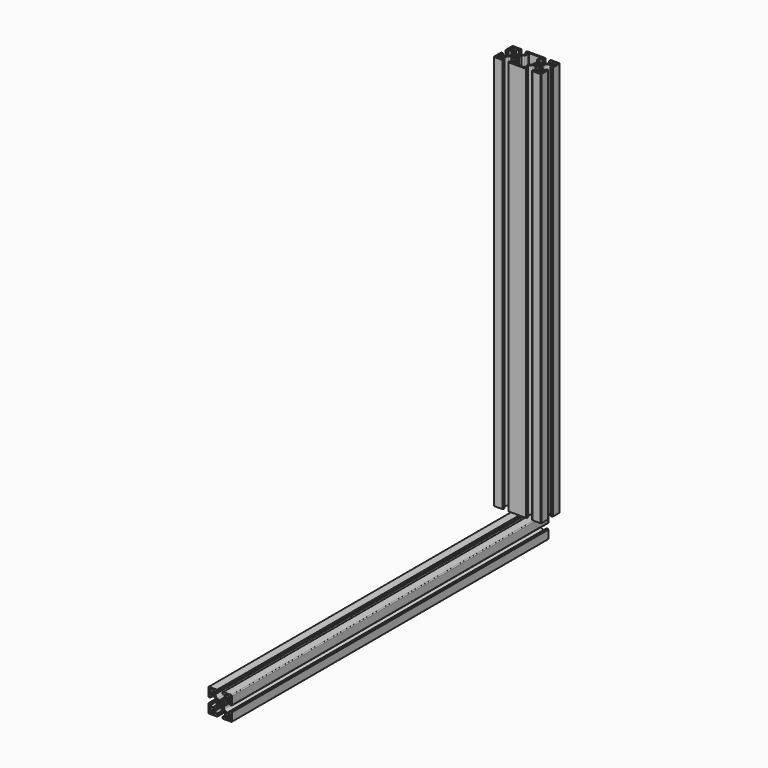
from build123d import *

# Parameters (mm, degrees)
F2_DEPTH = 500
F3_DEPTH = 500


# Not quite as in the source:
# - ends of sketch curves that miss each other by under 0.0002 mm in the source are joined


with BuildPart() as f2:
    # F1 (on Front) → F2 (new body)
    with BuildSketch(Plane.XZ):
        with BuildLine():
            Line((-16.817882, -28.053804), (-15.317882, -28.053804))
            ThreePointArc((-15.317882, -28.053804), (-15.2613573135, -27.5251941322), (-15.0943392862, -27.0204878701))
            ThreePointArc((-15.0943392862, -27.0204878701), (-15.1018556445, -26.757114112), (-15.3142900125, -26.6012490693))
            Line((-15.3142900125, -26.6012490693), (-16.055223, -26.467679))
            ThreePointArc((-16.055223, -26.467679), (-16.2747726412, -26.2973161033), (-16.2602657097, -26.0198001716))
            ThreePointArc((-16.2602657097, -26.0198001716), (-15.6451391247, -25.2265468753), (-14.8518861678, -24.611419716))
            ThreePointArc((-14.8518861678, -24.611419716), (-14.574370128, -24.5969122529), (-14.4040070693, -24.8164620125))
            Line((-14.4040070693, -24.8164620125), (-14.270436, -25.557396))
            ThreePointArc((-14.270436, -25.557396), (-14.114570705, -25.7698304515), (-13.8511966819, -25.7773467007))
            ThreePointArc((-13.8511966819, -25.7773467007), (-13.3464912208, -25.6103285465), (-12.817882, -25.553804))
            Line((-12.817882, -25.553804), (-12.817882, -24.053804))
            Line((-12.817882, -24.053804), (-13.317882, -23.553804))
            Line((-13.317882, -23.553804), (-15.035723, -23.553804))
            ThreePointArc((-15.035723, -23.553804), (-15.9762206131, -23.4025693887), (-16.8218943655, -22.9641134932))
            ThreePointArc((-16.8218943655, -22.9641134932), (-18.0925440917, -21.1637239049), (-18.9312372647, -19.1259440756))
            ThreePointArc((-18.9312372647, -19.1259440756), (-18.952848093, -18.864054156), (-18.9054896298, -18.6055767962))
            Line((-18.9054896298, -18.6055767962), (-17.917882, -15.553804))
            Line((-17.917882, -15.553804), (-16.267882, -15.553804))
            ThreePointArc((-16.267882, -15.553804), (-16.0557499656, -15.4659360344), (-15.967882, -15.253804))
            Line((-15.967882, -15.253804), (-15.967882, -13.553804))
            Line((-15.967882, -13.553804), (-16.767882, -13.053804))
            Line((-16.767882, -13.053804), (-26.817882, -13.053804))
            ThreePointArc((-26.817882, -13.053804), (-27.5249887812, -13.3466972188), (-27.817882, -14.053804))
            Line((-27.817882, -14.053804), (-27.817882, -24.103804))
            Line((-27.817882, -24.103804), (-27.317882, -24.903804))
            Line((-27.317882, -24.903804), (-25.617882, -24.903804))
            ThreePointArc((-25.617882, -24.903804), (-25.4057499656, -24.8159360344), (-25.317882, -24.603804))
            Line((-25.317882, -24.603804), (-25.317882, -22.953804))
            Line((-25.317882, -22.953804), (-22.266108, -21.966196))
            ThreePointArc((-22.266108, -21.966196), (-22.0076307271, -21.9188378518), (-21.7457409226, -21.9404486442))
            ThreePointArc((-21.7457409226, -21.9404486442), (-19.7079616374, -22.7791421598), (-17.907572504, -24.049791567))
            ThreePointArc((-17.907572504, -24.049791567), (-17.4691166439, -24.8954652882), (-17.317882, -25.835963))
            Line((-17.317882, -25.835963), (-17.317882, -27.553804))
            Line((-17.317882, -27.553804), (-16.817882, -28.053804))
        make_face()
        with BuildLine():
            ThreePointArc((-20.1318415243, -16.7176952608), (-19.817882, -18.053804), (-20.1318415243, -19.3899127392))
            ThreePointArc((-20.1318415243, -19.3899127392), (-20.1593135799, -19.5718836819), (-20.0753690344, -19.7356560344))
            Line((-20.0753690344, -19.7356560344), (-19.334799, -20.476227))
            ThreePointArc((-19.334799, -20.476227), (-19.2473630595, -20.6722640002), (-19.3132911489, -20.8765408801))
            ThreePointArc((-19.3132911489, -20.8765408801), (-19.6359009875, -21.2357840182), (-19.9951440617, -21.5583939234))
            ThreePointArc((-19.9951440617, -21.5583939234), (-20.1994212978, -21.6243229782), (-20.3954590344, -21.5368870344))
            Line((-20.3954590344, -21.5368870344), (-21.136029, -20.796316))
            ThreePointArc((-21.136029, -20.796316), (-21.2998015274, -20.7123715492), (-21.4817721923, -20.7398436134))
            ThreePointArc((-21.4817721923, -20.7398436134), (-22.8178815523, -21.053804), (-24.153991138, -20.7398442773))
            ThreePointArc((-24.153991138, -20.7398442773), (-24.3359616819, -20.7123714201), (-24.4997340344, -20.7963159656))
            Line((-24.4997340344, -20.7963159656), (-25.240304, -21.536887))
            ThreePointArc((-25.240304, -21.536887), (-25.4363417022, -21.6243229782), (-25.6406189751, -21.5583939691))
            ThreePointArc((-25.6406189751, -21.5583939691), (-25.9998625153, -21.2357845153), (-26.322472412, -20.8765413318))
            ThreePointArc((-26.322472412, -20.8765413318), (-26.3884009573, -20.6722643134), (-26.3009650344, -20.4762269656))
            Line((-26.3009650344, -20.4762269656), (-25.560394, -19.735656))
            ThreePointArc((-25.560394, -19.735656), (-25.4764494201, -19.5718836819), (-25.5039220121, -19.389913006))
            ThreePointArc((-25.5039220121, -19.389913006), (-25.817882, -18.053804), (-25.5039222773, -16.717694862))
            ThreePointArc((-25.5039222773, -16.717694862), (-25.4764494201, -16.5357243181), (-25.5603939656, -16.3719519656))
            Line((-25.5603939656, -16.3719519656), (-26.300965, -15.631381))
            ThreePointArc((-26.300965, -15.631381), (-26.3884009573, -15.4353436866), (-26.3224724576, -15.2310666314))
            ThreePointArc((-26.3224724576, -15.2310666314), (-25.9998625153, -14.8718234847), (-25.6406193318, -14.549213588))
            ThreePointArc((-25.6406193318, -14.549213588), (-25.4363417022, -14.4832850218), (-25.2403039656, -14.5707209656))
            Line((-25.2403039656, -14.5707209656), (-24.499734, -15.311292))
            ThreePointArc((-24.499734, -15.311292), (-24.3359616819, -15.3952365799), (-24.153991006, -15.3677639879))
            ThreePointArc((-24.153991006, -15.3677639879), (-22.8178815523, -15.053804), (-21.4817720604, -15.3677641214))
            ThreePointArc((-21.4817720604, -15.3677641214), (-21.2998015274, -15.3952364508), (-21.1360294656, -15.3112915344))
            Line((-21.1360294656, -15.3112915344), (-20.395459, -14.570721))
            ThreePointArc((-20.395459, -14.570721), (-20.1994212978, -14.4832850218), (-19.9951440249, -14.5492140309))
            ThreePointArc((-19.9951440249, -14.5492140309), (-19.6359009875, -14.8718239818), (-19.3132911946, -15.2310671567))
            ThreePointArc((-19.3132911946, -15.2310671567), (-19.2473630595, -15.4353439998), (-19.3347989656, -15.6313810344))
            Line((-19.3347989656, -15.6313810344), (-20.075369, -16.371952))
            ThreePointArc((-20.075369, -16.371952), (-20.1593135799, -16.5357243181), (-20.1318415243, -16.7176952608))
        make_face(mode=Mode.SUBTRACT)
        with BuildLine():
            Line((-10.317882, -28.053804), (-8.817882, -28.053804))
            Line((-8.817882, -28.053804), (-8.317882, -27.553804))
            Line((-8.317882, -27.553804), (-8.317882, -25.835963))
            ThreePointArc((-8.317882, -25.835963), (-8.1666472628, -24.8954650055), (-7.7281910149, -24.049790989))
            ThreePointArc((-7.7281910149, -24.049790989), (-5.9278016138, -22.7791417483), (-3.8900220756, -21.9404487353))
            ThreePointArc((-3.8900220756, -21.9404487353), (-3.6281322729, -21.9188378518), (-3.3696549943, -21.9661959825))
            Line((-3.3696549943, -21.9661959825), (-0.317882, -22.953804))
            Line((-0.317882, -22.953804), (-0.317882, -24.603804))
            ThreePointArc((-0.317882, -24.603804), (-0.2300140344, -24.8159360344), (-0.017882, -24.903804))
            Line((-0.017882, -24.903804), (1.682118, -24.903804))
            Line((1.682118, -24.903804), (2.182118, -24.103804))
            Line((2.182118, -24.103804), (2.182118, -14.053804))
            ThreePointArc((2.182118, -14.053804), (1.8892247812, -13.3466972188), (1.182118, -13.053804))
            Line((1.182118, -13.053804), (-8.867882, -13.053804))
            Line((-8.867882, -13.053804), (-9.667882, -13.553804))
            Line((-9.667882, -13.553804), (-9.667882, -15.253804))
            ThreePointArc((-9.667882, -15.253804), (-9.5800140344, -15.4659360344), (-9.367882, -15.553804))
            Line((-9.367882, -15.553804), (-7.717882, -15.553804))
            Line((-7.717882, -15.553804), (-6.730274, -18.605577))
            ThreePointArc((-6.730274, -18.605577), (-6.6829159047, -18.8640542036), (-6.7045263914, -19.1259439149))
            ThreePointArc((-6.7045263914, -19.1259439149), (-7.5432189083, -21.1637239049), (-8.8138685119, -22.9641134339))
            ThreePointArc((-8.8138685119, -22.9641134339), (-9.6595430055, -23.4025692628), (-10.600041, -23.553804))
            Line((-10.600041, -23.553804), (-12.317882, -23.553804))
            Line((-12.317882, -23.553804), (-12.817882, -24.053804))
            Line((-12.817882, -24.053804), (-12.817882, -25.553804))
            ThreePointArc((-12.817882, -25.553804), (-12.2892723342, -25.6103286428), (-11.7845662465, -25.777346543))
            ThreePointArc((-11.7845662465, -25.777346543), (-11.521192295, -25.7698304515), (-11.3653270693, -25.5573959875))
            Line((-11.3653270693, -25.5573959875), (-11.231756, -24.816462))
            ThreePointArc((-11.231756, -24.816462), (-11.061392872, -24.5969122529), (-10.7838767336, -24.6114195492))
            ThreePointArc((-10.7838767336, -24.6114195492), (-9.990624391, -25.2265473595), (-9.3754974572, -26.0198002702))
            ThreePointArc((-9.3754974572, -26.0198002702), (-9.3609903588, -26.2973161033), (-9.5805400125, -26.4676789307))
            Line((-9.5805400125, -26.4676789307), (-10.321473, -26.601249))
            ThreePointArc((-10.321473, -26.601249), (-10.5339073555, -26.757114112), (-10.5414238716, -27.0204879417))
            ThreePointArc((-10.5414238716, -27.0204879417), (-10.3744066428, -27.5251943342), (-10.317882, -28.053804))
        make_face()
        with BuildLine():
            ThreePointArc((-5.5627339656, -19.7356560344), (-5.4787894201, -19.5718836819), (-5.5062620121, -19.389913006))
            ThreePointArc((-5.5062620121, -19.389913006), (-5.820221, -18.053804), (-5.5062614757, -16.7176952608))
            ThreePointArc((-5.5062614757, -16.7176952608), (-5.4787894201, -16.5357243181), (-5.5627339656, -16.3719519656))
            Line((-5.5627339656, -16.3719519656), (-6.303305, -15.631381))
            ThreePointArc((-6.303305, -15.631381), (-6.3907399595, -15.4353436467), (-6.3248118511, -15.2310671199))
            ThreePointArc((-6.3248118511, -15.2310671199), (-6.0022020125, -14.8718239818), (-5.6429589383, -14.5492140766))
            ThreePointArc((-5.6429589383, -14.5492140766), (-5.4386817022, -14.4832850218), (-5.2426439656, -14.5707209656))
            Line((-5.2426439656, -14.5707209656), (-4.502074, -15.311292))
            ThreePointArc((-4.502074, -15.311292), (-4.3383016819, -15.3952365799), (-4.156331006, -15.3677639879))
            ThreePointArc((-4.156331006, -15.3677639879), (-2.8202214477, -15.053804), (-1.484111862, -15.3677637227))
            ThreePointArc((-1.484111862, -15.3677637227), (-1.3021413181, -15.3952365799), (-1.1383689656, -15.3112920344))
            Line((-1.1383689656, -15.3112920344), (-0.397799, -14.570721))
            ThreePointArc((-0.397799, -14.570721), (-0.2017612978, -14.4832850218), (0.0025159751, -14.5492140309))
            ThreePointArc((0.0025159751, -14.5492140309), (0.3617595153, -14.8718234847), (0.684369412, -15.2310666682))
            ThreePointArc((0.684369412, -15.2310666682), (0.7502979573, -15.4353436866), (0.6628620344, -15.6313810344))
            Line((0.6628620344, -15.6313810344), (-0.077709, -16.371952))
            ThreePointArc((-0.077709, -16.371952), (-0.1616535799, -16.5357243181), (-0.1341809879, -16.717694994))
            ThreePointArc((-0.1341809879, -16.717694994), (0.179779, -18.053804), (-0.1341807227, -19.389913138))
            ThreePointArc((-0.1341807227, -19.389913138), (-0.1616535799, -19.5718836819), (-0.0777090344, -19.7356560344))
            Line((-0.0777090344, -19.7356560344), (0.662862, -20.476227))
            ThreePointArc((0.662862, -20.476227), (0.7502979573, -20.6722643134), (0.6843694576, -20.8765413686))
            ThreePointArc((0.6843694576, -20.8765413686), (0.3617595153, -21.2357845153), (0.0025163318, -21.558394412))
            ThreePointArc((0.0025163318, -21.558394412), (-0.2017612978, -21.6243229782), (-0.3977990344, -21.5368870344))
            Line((-0.3977990344, -21.5368870344), (-1.138369, -20.796316))
            ThreePointArc((-1.138369, -20.796316), (-1.3021413181, -20.7123714201), (-1.484111994, -20.7398440121))
            ThreePointArc((-1.484111994, -20.7398440121), (-2.8202214477, -21.053804), (-4.1563309396, -20.7398438786))
            ThreePointArc((-4.1563309396, -20.7398438786), (-4.3383016819, -20.7123714201), (-4.5020740344, -20.7963159656))
            Line((-4.5020740344, -20.7963159656), (-5.242644, -21.536887))
            ThreePointArc((-5.242644, -21.536887), (-5.4386817022, -21.6243229782), (-5.6429589751, -21.5583939691))
            ThreePointArc((-5.6429589751, -21.5583939691), (-6.0022020125, -21.2357840182), (-6.3248118054, -20.8765408433))
            ThreePointArc((-6.3248118054, -20.8765408433), (-6.3907399595, -20.6722643533), (-6.3033045344, -20.4762274656))
            Line((-6.3033045344, -20.4762274656), (-5.5627339656, -19.7356560344))
        make_face(mode=Mode.SUBTRACT)
        with BuildLine():
            Line((-8.317882, -28.553804), (-8.817882, -28.053804))
            Line((-8.817882, -28.053804), (-10.317882, -28.053804))
            ThreePointArc((-10.317882, -28.053804), (-10.3744066428, -28.5824136658), (-10.541424543, -29.0871197535))
            ThreePointArc((-10.541424543, -29.0871197535), (-10.5339073967, -29.3504938095), (-10.3214731621, -29.5063588992))
            Line((-10.3214731621, -29.5063588992), (-9.58054, -29.639929))
            ThreePointArc((-9.58054, -29.639929), (-9.3609903588, -29.8102918967), (-9.3754972903, -30.0878078284))
            ThreePointArc((-9.3754972903, -30.0878078284), (-9.990624391, -30.8810606405), (-10.783877091, -31.496187846))
            ThreePointArc((-10.783877091, -31.496187846), (-11.061392872, -31.5106957471), (-11.2317559307, -31.2911459875))
            Line((-11.2317559307, -31.2911459875), (-11.365327, -30.550212))
            ThreePointArc((-11.365327, -30.550212), (-11.521192112, -30.3377776445), (-11.7845659417, -30.3302611284))
            ThreePointArc((-11.7845659417, -30.3302611284), (-12.2892721322, -30.4972793135), (-12.817882, -30.553804))
            Line((-12.817882, -30.553804), (-12.817882, -32.053804))
            Line((-12.817882, -32.053804), (-12.317882, -32.553804))
            Line((-12.317882, -32.553804), (-10.600041, -32.553804))
            ThreePointArc((-10.600041, -32.553804), (-9.6595430055, -32.7050387372), (-8.813868989, -33.1434949851))
            ThreePointArc((-8.813868989, -33.1434949851), (-7.5432189083, -34.9438840951), (-6.7045257353, -36.9816639244))
            ThreePointArc((-6.7045257353, -36.9816639244), (-6.6829158812, -37.2435533212), (-6.7302739825, -37.5020300057))
            Line((-6.7302739825, -37.5020300057), (-7.717882, -40.553804))
            Line((-7.717882, -40.553804), (-9.367882, -40.553804))
            ThreePointArc((-9.367882, -40.553804), (-9.5800140344, -40.6416719656), (-9.667882, -40.853804))
            Line((-9.667882, -40.853804), (-9.667882, -42.553804))
            Line((-9.667882, -42.553804), (-8.867882, -43.053804))
            Line((-8.867882, -43.053804), (1.182118, -43.053804))
            ThreePointArc((1.182118, -43.053804), (1.8892247812, -42.7609107812), (2.182118, -42.053804))
            Line((2.182118, -42.053804), (2.182118, -32.003804))
            Line((2.182118, -32.003804), (1.682118, -31.203804))
            Line((1.682118, -31.203804), (-0.017882, -31.203804))
            ThreePointArc((-0.017882, -31.203804), (-0.2300140344, -31.2916719656), (-0.317882, -31.503804))
            Line((-0.317882, -31.503804), (-0.317882, -33.153804))
            Line((-0.317882, -33.153804), (-3.369655, -34.141412))
            ThreePointArc((-3.369655, -34.141412), (-3.6281322729, -34.1887701482), (-3.8900220774, -34.1671593558))
            ThreePointArc((-3.8900220774, -34.1671593558), (-5.9278016138, -33.3284662517), (-7.7281909374, -32.0578169295))
            ThreePointArc((-7.7281909374, -32.0578169295), (-8.1666472628, -31.2121429945), (-8.317882, -30.271645))
            Line((-8.317882, -30.271645), (-8.317882, -28.553804))
        make_face()
        with BuildLine():
            ThreePointArc((-5.507146239, -39.3904841188), (-5.8210019909, -38.0543501064), (-5.5069379006, -36.7182650494))
            ThreePointArc((-5.5069379006, -36.7182650494), (-5.4794506299, -36.5362965287), (-5.5633824662, -36.3725174663))
            Line((-5.5633824662, -36.3725174663), (-6.303896, -35.631889))
            ThreePointArc((-6.303896, -35.631889), (-6.3913162338, -35.4358449105), (-6.3253716664, -35.2315732687))
            ThreePointArc((-6.3253716664, -35.2315732687), (-6.0027340882, -34.8723550769), (-5.6434657786, -34.5497732749))
            ThreePointArc((-5.6434657786, -34.5497732749), (-5.4391833549, -34.483860277), (-5.2431524662, -34.5713114663))
            Line((-5.2431524662, -34.5713114663), (-4.50264, -35.31194))
            ThreePointArc((-4.50264, -35.31194), (-4.3388740212, -35.3958977668), (-4.1569008286, -35.3684393446))
            ThreePointArc((-4.1569008286, -35.3684393446), (-2.8207674361, -35.0545840092), (-1.4846830494, -35.3686480994))
            ThreePointArc((-1.4846830494, -35.3686480994), (-1.3027146578, -35.3961343911), (-1.1389359663, -35.3122030337))
            Line((-1.1389359663, -35.3122030337), (-0.398307, -34.57169))
            ThreePointArc((-0.398307, -34.57169), (-0.2022626922, -34.4842688081), (0.0020096134, -34.5502132386))
            ThreePointArc((0.0020096134, -34.5502132386), (0.3612269231, -34.8728519118), (0.6838087251, -35.2321202214))
            ThreePointArc((0.6838087251, -35.2321202214), (0.7497216831, -35.4364023869), (0.6622700337, -35.6324330337))
            Line((0.6622700337, -35.6324330337), (-0.078358, -36.372946))
            ThreePointArc((-0.078358, -36.372946), (-0.1623158238, -36.5367113277), (-0.1348573446, -36.7186841714))
            ThreePointArc((-0.1348573446, -36.7186841714), (0.1789979909, -38.0548178935), (-0.1350659009, -39.3909025518))
            ThreePointArc((-0.1350659009, -39.3909025518), (-0.162552241, -39.5728712621), (-0.0786200338, -39.7366500338))
            Line((-0.0786200338, -39.7366500338), (0.661893, -40.477278))
            ThreePointArc((0.661893, -40.477278), (0.7493132149, -40.6733227364), (0.6833686664, -40.8775947313))
            ThreePointArc((0.6833686664, -40.8775947313), (0.3607308072, -41.2368122042), (0.0014628737, -41.5593938432))
            ThreePointArc((0.0014628737, -41.5593938432), (-0.202819292, -41.625306742), (-0.3988500338, -41.5378560338))
            Line((-0.3988500338, -41.5378560338), (-1.139363, -40.797227))
            ThreePointArc((-1.139363, -40.797227), (-1.303129108, -40.7132702121), (-1.4851017727, -40.7407284571))
            ThreePointArc((-1.4851017727, -40.7407284571), (-2.8212354459, -41.0545839909), (-4.157320149, -40.7405202994))
            ThreePointArc((-4.157320149, -40.7405202994), (-4.3392886912, -40.7130336658), (-4.5030675338, -40.7969654663))
            Line((-4.5030675338, -40.7969654663), (-5.243696, -41.537478))
            ThreePointArc((-5.243696, -41.537478), (-5.4397403476, -41.624898194), (-5.6440121248, -41.5589541549))
            ThreePointArc((-5.6440121248, -41.5589541549), (-6.0032304261, -41.2363165853), (-6.3258123317, -40.8770482671))
            ThreePointArc((-6.3258123317, -40.8770482671), (-6.3917246831, -40.6727656131), (-6.3042730337, -40.4767349663))
            Line((-6.3042730337, -40.4767349663), (-5.563645, -39.736222))
            ThreePointArc((-5.563645, -39.736222), (-5.4796873054, -39.5724564631), (-5.507146239, -39.3904841188))
        make_face(mode=Mode.SUBTRACT)
        with BuildLine():
            ThreePointArc((-15.0943392862, -29.0871201299), (-15.2613573135, -28.5824138678), (-15.317882, -28.053804))
            Line((-15.317882, -28.053804), (-16.817882, -28.053804))
            Line((-16.817882, -28.053804), (-17.317882, -28.553804))
            Line((-17.317882, -28.553804), (-17.317882, -30.271645))
            ThreePointArc((-17.317882, -30.271645), (-17.4691166439, -31.2121427118), (-17.9075726307, -32.0578165326))
            ThreePointArc((-17.9075726307, -32.0578165326), (-19.7079616374, -33.3284658402), (-21.7457409999, -34.1671590005))
            ThreePointArc((-21.7457409999, -34.1671590005), (-22.0076307271, -34.1887701482), (-22.2661080057, -34.1414120175))
            Line((-22.2661080057, -34.1414120175), (-25.317882, -33.153804))
            Line((-25.317882, -33.153804), (-25.317882, -31.503804))
            ThreePointArc((-25.317882, -31.503804), (-25.4057499656, -31.2916719656), (-25.617882, -31.203804))
            Line((-25.617882, -31.203804), (-27.317882, -31.203804))
            Line((-27.317882, -31.203804), (-27.817882, -32.003804))
            Line((-27.817882, -32.003804), (-27.817882, -42.053804))
            ThreePointArc((-27.817882, -42.053804), (-27.5249887812, -42.7609107812), (-26.817882, -43.053804))
            Line((-26.817882, -43.053804), (-16.767882, -43.053804))
            Line((-16.767882, -43.053804), (-15.967882, -42.553804))
            Line((-15.967882, -42.553804), (-15.967882, -40.853804))
            ThreePointArc((-15.967882, -40.853804), (-16.0557499656, -40.6416719656), (-16.267882, -40.553804))
            Line((-16.267882, -40.553804), (-17.917882, -40.553804))
            Line((-17.917882, -40.553804), (-18.905489, -37.50203))
            ThreePointArc((-18.905489, -37.50203), (-18.9528481165, -37.2435533689), (-18.9312375634, -36.9816638775))
            ThreePointArc((-18.9312375634, -36.9816638775), (-18.0925440917, -34.9438840951), (-16.8218944881, -33.1434945661))
            ThreePointArc((-16.8218944881, -33.1434945661), (-15.9762206131, -32.7050386113), (-15.035723, -32.553804))
            Line((-15.035723, -32.553804), (-13.317882, -32.553804))
            Line((-13.317882, -32.553804), (-12.817882, -32.053804))
            Line((-12.817882, -32.053804), (-12.817882, -30.553804))
            ThreePointArc((-12.817882, -30.553804), (-13.3464914228, -30.4972794098), (-13.8511973007, -30.3302616625))
            ThreePointArc((-13.8511973007, -30.3302616625), (-14.114570888, -30.3377776445), (-14.2704359307, -30.5502120125))
            Line((-14.2704359307, -30.5502120125), (-14.404007, -31.291146))
            ThreePointArc((-14.404007, -31.291146), (-14.574370128, -31.5106957471), (-14.8518862664, -31.4961884508))
            ThreePointArc((-14.8518862664, -31.4961884508), (-15.6451391247, -30.8810611247), (-16.260266284, -30.0878081678))
            ThreePointArc((-16.260266284, -30.0878081678), (-16.2747726412, -29.8102918967), (-16.0552229875, -29.6399290693))
            Line((-16.0552229875, -29.6399290693), (-15.31429, -29.506358))
            ThreePointArc((-15.31429, -29.506358), (-15.1018556033, -29.3504938095), (-15.0943392862, -29.0871201299))
        make_face()
        with BuildLine():
            ThreePointArc((-20.0747205338, -36.3725174663), (-20.1586523342, -36.5362963089), (-20.1311656295, -36.7182648157))
            ThreePointArc((-20.1311656295, -36.7182648157), (-19.8171020091, -38.0543498837), (-20.1309575628, -39.3904837201))
            ThreePointArc((-20.1309575628, -39.3904837201), (-20.1584156946, -39.5724564631), (-20.0744580337, -39.7362220337))
            Line((-20.0744580337, -39.7362220337), (-19.33383, -40.476735))
            ThreePointArc((-19.33383, -40.476735), (-19.2463783169, -40.6727656131), (-19.3122908476, -40.8770481227))
            ThreePointArc((-19.3122908476, -40.8770481227), (-19.6348730769, -41.2363160882), (-19.9940910142, -41.5589539824))
            ThreePointArc((-19.9940910142, -41.5589539824), (-20.1983629105, -41.6248982338), (-20.3944070337, -41.5374780337))
            Line((-20.3944070337, -41.5374780337), (-21.135036, -40.796965))
            ThreePointArc((-21.135036, -40.796965), (-21.2988146578, -40.7130336089), (-21.4807828157, -40.7405203705))
            ThreePointArc((-21.4807828157, -40.7405203705), (-22.8168676587, -41.0545839908), (-24.1530013171, -40.7407286377))
            ThreePointArc((-24.1530013171, -40.7407286377), (-24.334973892, -40.7132702121), (-24.4987395337, -40.7972274662))
            Line((-24.4987395337, -40.7972274662), (-25.239253, -41.537856))
            ThreePointArc((-25.239253, -41.537856), (-25.435283708, -41.625306742), (-25.6395657293, -41.5593936639))
            ThreePointArc((-25.6395657293, -41.5593936639), (-25.99883431, -41.2368127014), (-26.3214719824, -40.8775949858))
            ThreePointArc((-26.3214719824, -40.8775949858), (-26.3874162149, -40.6733227364), (-26.2999955337, -40.4772784662))
            Line((-26.2999955337, -40.4772784662), (-25.559483, -39.73665))
            ThreePointArc((-25.559483, -39.73665), (-25.475550759, -39.5728712621), (-25.5030371701, -39.3909025871))
            ThreePointArc((-25.5030371701, -39.3909025871), (-25.8171019909, -38.0548178936), (-25.503246239, -36.7186838812))
            ThreePointArc((-25.503246239, -36.7186838812), (-25.4757871762, -36.5367113277), (-25.5597444663, -36.3729454662))
            Line((-25.5597444663, -36.3729454662), (-26.300374, -35.632433))
            ThreePointArc((-26.300374, -35.632433), (-26.3878247021, -35.4364020339), (-26.3219121524, -35.2321198773))
            ThreePointArc((-26.3219121524, -35.2321198773), (-25.9993304261, -34.8728514147), (-25.6401123794, -34.550213529))
            ThreePointArc((-25.6401123794, -34.550213529), (-25.4358403078, -34.4842688081), (-25.2397959662, -34.5716899662))
            Line((-25.2397959662, -34.5716899662), (-24.499168, -35.312203))
            ThreePointArc((-24.499168, -35.312203), (-24.3353886912, -35.3961343342), (-24.1534201843, -35.3686476295))
            ThreePointArc((-24.1534201843, -35.3686476295), (-22.8173356686, -35.0545840091), (-21.4812022799, -35.3684395628))
            ThreePointArc((-21.4812022799, -35.3684395628), (-21.2992289788, -35.3958977668), (-21.1354629663, -35.3119400337))
            Line((-21.1354629663, -35.3119400337), (-20.39495, -34.571312))
            ThreePointArc((-20.39495, -34.571312), (-20.1989200339, -34.4838602979), (-19.9946378773, -34.5497728476))
            ThreePointArc((-19.9946378773, -34.5497728476), (-19.63536969, -34.8723552987), (-19.312731624, -35.2315735027))
            ThreePointArc((-19.312731624, -35.2315735027), (-19.2467867662, -35.4358449105), (-19.3342069663, -35.6318890337))
            Line((-19.3342069663, -35.6318890337), (-20.0747205338, -36.3725174663))
        make_face(mode=Mode.SUBTRACT)
    extrude(amount=F2_DEPTH)


with BuildPart() as f3:
    # F0 (on Top) → F3 (new body)
    with BuildSketch(Plane.XY):
        with BuildLine():
            ThreePointArc((13.887110457, -26.0471442465), (14.0541283572, -26.5518503342), (14.110653, -27.08046))
            Line((14.110653, -27.08046), (15.610653, -27.08046))
            Line((15.610653, -27.08046), (16.110653, -26.58046))
            Line((16.110653, -26.58046), (16.110653, -24.862619))
            ThreePointArc((16.110653, -24.862619), (16.2618877372, -23.9221210055), (16.7003439851, -23.076446989))
            ThreePointArc((16.7003439851, -23.076446989), (18.5007333862, -21.8057977483), (20.5385129244, -20.9671047353))
            ThreePointArc((20.5385129244, -20.9671047353), (20.8004026903, -20.9454938994), (21.0588799109, -20.9928522754))
            Line((21.0588799109, -20.9928522754), (24.110653, -21.98046))
            Line((24.110653, -21.98046), (24.110653, -23.63046))
            ThreePointArc((24.110653, -23.63046), (24.1985209656, -23.8425920344), (24.410653, -23.93046))
            Line((24.410653, -23.93046), (26.110653, -23.93046))
            Line((26.110653, -23.93046), (26.610653, -23.13046))
            Line((26.610653, -23.13046), (26.610653, -13.08046))
            ThreePointArc((26.610653, -13.08046), (26.3177597812, -12.3733532188), (25.610653, -12.08046))
            Line((25.610653, -12.08046), (15.560653, -12.08046))
            Line((15.560653, -12.08046), (14.760653, -12.58046))
            Line((14.760653, -12.58046), (14.760653, -14.28046))
            ThreePointArc((14.760653, -14.28046), (14.8485209656, -14.4925920344), (15.060653, -14.58046))
            Line((15.060653, -14.58046), (16.710653, -14.58046))
            Line((16.710653, -14.58046), (17.698261, -17.632234))
            ThreePointArc((17.698261, -17.632234), (17.7456191188, -17.8907106788), (17.7240086086, -18.1525999149))
            ThreePointArc((17.7240086086, -18.1525999149), (16.8853153179, -20.1903794934), (15.6146659295, -21.9907689374))
            ThreePointArc((15.6146659295, -21.9907689374), (14.7689919945, -22.4292252628), (13.828494, -22.58046))
            Line((13.828494, -22.58046), (12.110653, -22.58046))
            Line((12.110653, -22.58046), (11.610653, -23.08046))
            Line((11.610653, -23.08046), (11.610653, -24.58046))
            ThreePointArc((11.610653, -24.58046), (12.1392628678, -24.6369846865), (12.6439691299, -24.8040027138))
            ThreePointArc((12.6439691299, -24.8040027138), (12.907342888, -24.7964863555), (13.0632079307, -24.5840519875))
            Line((13.0632079307, -24.5840519875), (13.196778, -23.843118))
            ThreePointArc((13.196778, -23.843118), (13.367141128, -23.6235682529), (13.6446572664, -23.6380755492))
            ThreePointArc((13.6446572664, -23.6380755492), (14.4379103046, -24.2532030551), (15.0530375428, -25.0464562702))
            ThreePointArc((15.0530375428, -25.0464562702), (15.0675446412, -25.3239721033), (14.8479949875, -25.4943349307))
            Line((14.8479949875, -25.4943349307), (14.107061, -25.627906))
            ThreePointArc((14.107061, -25.627906), (13.8946276274, -25.7837711445), (13.887110457, -26.0471442465))
        make_face()
        with BuildLine():
            ThreePointArc((18.8658010344, -18.7623120344), (18.9497455799, -18.5985396819), (18.9222729879, -18.416569006))
            ThreePointArc((18.9222729879, -18.416569006), (18.608313, -17.08046), (18.9222727227, -15.744350862))
            ThreePointArc((18.9222727227, -15.744350862), (18.9497455799, -15.5623803181), (18.8658010344, -15.3986079656))
            Line((18.8658010344, -15.3986079656), (18.12523, -14.658037))
            ThreePointArc((18.12523, -14.658037), (18.0377940427, -14.4619996866), (18.1037225424, -14.2577226314))
            ThreePointArc((18.1037225424, -14.2577226314), (18.4263324847, -13.8984794847), (18.7855756682, -13.575869588))
            ThreePointArc((18.7855756682, -13.575869588), (18.9898526866, -13.5099410427), (19.1858900344, -13.5973769656))
            Line((19.1858900344, -13.5973769656), (19.926461, -14.337948))
            ThreePointArc((19.926461, -14.337948), (20.0902333181, -14.4218925799), (20.272203994, -14.3944199879))
            ThreePointArc((20.272203994, -14.3944199879), (21.608313, -14.08046), (22.944422138, -14.3944197227))
            ThreePointArc((22.944422138, -14.3944197227), (23.1263926819, -14.4218925799), (23.2901650344, -14.3379480344))
            Line((23.2901650344, -14.3379480344), (24.030736, -13.597377))
            ThreePointArc((24.030736, -13.597377), (24.2267737022, -13.5099410218), (24.4310509751, -13.5758700309))
            ThreePointArc((24.4310509751, -13.5758700309), (24.7902940125, -13.8984799818), (25.1129038054, -14.2577231567))
            ThreePointArc((25.1129038054, -14.2577231567), (25.1788319405, -14.4619999998), (25.0913960344, -14.6580370344))
            Line((25.0913960344, -14.6580370344), (24.350826, -15.398608))
            ThreePointArc((24.350826, -15.398608), (24.2668814201, -15.5623803181), (24.2943540121, -15.744350994))
            ThreePointArc((24.2943540121, -15.744350994), (24.608313, -17.08046), (24.2943534757, -18.4165687392))
            ThreePointArc((24.2943534757, -18.4165687392), (24.2668814201, -18.5985396819), (24.3508259656, -18.7623120344))
            Line((24.3508259656, -18.7623120344), (25.091396, -19.502883))
            ThreePointArc((25.091396, -19.502883), (25.1788319614, -19.6989203891), (25.1129033626, -19.9031974866))
            ThreePointArc((25.1129033626, -19.9031974866), (24.7902935153, -20.2624405153), (24.4310504498, -20.5850503169))
            ThreePointArc((24.4310504498, -20.5850503169), (24.2267733891, -20.6509789614), (24.0307359656, -20.5635430344))
            Line((24.0307359656, -20.5635430344), (23.290165, -19.822972))
            ThreePointArc((23.290165, -19.822972), (23.1263925527, -19.739028399), (22.9444224048, -19.7665008138))
            ThreePointArc((22.9444224048, -19.7665008138), (21.608313, -20.08046), (20.272203862, -19.7665002773))
            ThreePointArc((20.272203862, -19.7665002773), (20.0902334473, -19.739028399), (19.9264614656, -19.8229724656))
            Line((19.9264614656, -19.8229724656), (19.18589, -20.563543))
            ThreePointArc((19.18589, -20.563543), (18.9898529998, -20.6509789405), (18.7855761199, -20.5850508511))
            ThreePointArc((18.7855761199, -20.5850508511), (18.4263329818, -20.2624410125), (18.1037230766, -19.9031979383))
            ThreePointArc((18.1037230766, -19.9031979383), (18.0377940218, -19.6989207022), (18.1252299656, -19.5028829656))
            Line((18.1252299656, -19.5028829656), (18.8658010344, -18.7623120344))
        make_face(mode=Mode.SUBTRACT)
        with BuildLine():
            Line((15.610653, -27.08046), (14.110653, -27.08046))
            ThreePointArc((14.110653, -27.08046), (14.0541283572, -27.6090696658), (13.887110457, -28.1137757535))
            ThreePointArc((13.887110457, -28.1137757535), (13.8946274159, -28.3771494523), (14.107061044, -28.5330147561))
            Line((14.107061044, -28.5330147561), (14.847995, -28.666585))
            ThreePointArc((14.847995, -28.666585), (15.0675446412, -28.8369478967), (15.0530377097, -29.1144638284))
            ThreePointArc((15.0530377097, -29.1144638284), (14.4379101247, -29.9077171247), (13.6446567298, -30.5228445428))
            ThreePointArc((13.6446567298, -30.5228445428), (13.3671408967, -30.5373516412), (13.1967780693, -30.3178019875))
            Line((13.1967780693, -30.3178019875), (13.063208, -29.576868))
            ThreePointArc((13.063208, -29.576868), (12.9073424523, -29.3644344159), (12.6439690583, -29.3569181284))
            ThreePointArc((12.6439690583, -29.3569181284), (12.1392626658, -29.5239353572), (11.610653, -29.58046))
            Line((11.610653, -29.58046), (11.610653, -31.08046))
            Line((11.610653, -31.08046), (12.110653, -31.58046))
            Line((12.110653, -31.58046), (13.828494, -31.58046))
            ThreePointArc((13.828494, -31.58046), (14.7689919945, -31.7316947372), (15.614666011, -32.1701509851))
            ThreePointArc((15.614666011, -32.1701509851), (16.8853153179, -33.9705405066), (17.7240083402, -36.0083201886))
            ThreePointArc((17.7240083402, -36.0083201886), (17.7456190953, -36.2702097964), (17.6982607246, -36.5286869109))
            Line((17.6982607246, -36.5286869109), (16.710653, -39.58046))
            Line((16.710653, -39.58046), (15.060653, -39.58046))
            ThreePointArc((15.060653, -39.58046), (14.8485209656, -39.6683279656), (14.760653, -39.88046))
            Line((14.760653, -39.88046), (14.760653, -41.58046))
            Line((14.760653, -41.58046), (15.560653, -42.08046))
            Line((15.560653, -42.08046), (25.610653, -42.08046))
            ThreePointArc((25.610653, -42.08046), (26.3177597812, -41.7875667812), (26.610653, -41.08046))
            Line((26.610653, -41.08046), (26.610653, -31.03046))
            Line((26.610653, -31.03046), (26.110653, -30.23046))
            Line((26.110653, -30.23046), (24.410653, -30.23046))
            ThreePointArc((24.410653, -30.23046), (24.1985209656, -30.3183279656), (24.110653, -30.53046))
            Line((24.110653, -30.53046), (24.110653, -32.18046))
            Line((24.110653, -32.18046), (21.05888, -33.168068))
            ThreePointArc((21.05888, -33.168068), (20.8004027964, -33.2154260953), (20.5385130851, -33.1938156086))
            ThreePointArc((20.5385130851, -33.1938156086), (18.5007330951, -32.3551230917), (16.7003435661, -31.0844734881))
            ThreePointArc((16.7003435661, -31.0844734881), (16.2618877372, -30.2387989945), (16.110653, -29.298301))
            Line((16.110653, -29.298301), (16.110653, -27.58046))
            Line((16.110653, -27.58046), (15.610653, -27.08046))
        make_face()
        with BuildLine():
            ThreePointArc((18.921388761, -38.4171401188), (18.6075330091, -37.0810065541), (18.9215967006, -35.744921851))
            ThreePointArc((18.9215967006, -35.744921851), (18.9490843131, -35.5629531797), (18.8651520338, -35.3991739662))
            Line((18.8651520338, -35.3991739662), (18.124639, -34.658546))
            ThreePointArc((18.124639, -34.658546), (18.0372187851, -34.4625012636), (18.1031633336, -34.2582292687))
            ThreePointArc((18.1031633336, -34.2582292687), (18.42580069, -33.8990112986), (18.7850687329, -33.5764296683))
            ThreePointArc((18.7850687329, -33.5764296683), (18.989351292, -33.510517258), (19.1853820338, -33.5979679662))
            Line((19.1853820338, -33.5979679662), (19.925895, -34.338597))
            ThreePointArc((19.925895, -34.338597), (20.089661108, -34.4225537879), (20.2716337727, -34.3950955429))
            ThreePointArc((20.2716337727, -34.3950955429), (21.6077673413, -34.0812400092), (22.9438519506, -34.3953040994))
            ThreePointArc((22.9438519506, -34.3953040994), (23.1258204713, -34.4227913701), (23.2895995337, -34.3388595338))
            Line((23.2895995337, -34.3388595338), (24.030228, -33.598346))
            ThreePointArc((24.030228, -33.598346), (24.2262720895, -33.5109257662), (24.4305437313, -33.5768703336))
            ThreePointArc((24.4305437313, -33.5768703336), (24.7897619231, -33.8995079118), (25.1123437251, -34.2587762214))
            ThreePointArc((25.1123437251, -34.2587762214), (25.1782566831, -34.4630583869), (25.0908050337, -34.6590890337))
            Line((25.0908050337, -34.6590890337), (24.350177, -35.399602))
            ThreePointArc((24.350177, -35.399602), (24.2662192332, -35.5633679788), (24.2936776554, -35.7453411714))
            ThreePointArc((24.2936776554, -35.7453411714), (24.6075329908, -37.0814745639), (24.2934689006, -38.4175589506))
            ThreePointArc((24.2934689006, -38.4175589506), (24.2659826089, -38.5995273422), (24.3499139663, -38.7633060337))
            Line((24.3499139663, -38.7633060337), (25.090427, -39.503935))
            ThreePointArc((25.090427, -39.503935), (25.1778482317, -39.6999790497), (25.1119032729, -39.9042512198))
            ThreePointArc((25.1119032729, -39.9042512198), (24.7892650882, -40.2634689231), (24.4299967786, -40.5860507251))
            ThreePointArc((24.4299967786, -40.5860507251), (24.2257146131, -40.6519636831), (24.0296839663, -40.5645120337))
            Line((24.0296839663, -40.5645120337), (23.289171, -39.823884))
            ThreePointArc((23.289171, -39.823884), (23.1254056723, -39.7399261762), (22.9434328286, -39.7673846554))
            ThreePointArc((22.9434328286, -39.7673846554), (21.6072993314, -40.0812399909), (20.271214851, -39.7671762994))
            ThreePointArc((20.271214851, -39.7671762994), (20.0892463088, -39.7396896658), (19.9254674662, -39.8236214663))
            Line((19.9254674662, -39.8236214663), (19.184839, -40.564134))
            ThreePointArc((19.184839, -40.564134), (18.9887946922, -40.6515551919), (18.7845223866, -40.5856107614))
            ThreePointArc((18.7845223866, -40.5856107614), (18.4253045739, -40.2629725853), (18.1027226683, -39.9037042671))
            ThreePointArc((18.1027226683, -39.9037042671), (18.0368102979, -39.6994219661), (18.1242614662, -39.5033914663))
            Line((18.1242614662, -39.5033914663), (18.86489, -38.762878))
            ThreePointArc((18.86489, -38.762878), (18.948846845, -38.5991125431), (18.921388761, -38.4171401188))
        make_face(mode=Mode.SUBTRACT)
        with BuildLine():
            Line((9.110653, -27.08046), (7.110653, -27.08046))
            Line((7.110653, -27.08046), (6.610653, -27.58046))
            Line((6.610653, -27.58046), (6.610653, -31.094338))
            ThreePointArc((6.610653, -31.094338), (6.5757763325, -31.2778053964), (6.4760118579, -31.4356778672))
            Line((6.4760118579, -31.4356778672), (4.687781, -33.349742))
            ThreePointArc((4.687781, -33.349742), (3.7034336778, -35.2239337785), (3.8134822947, -37.3380349024))
            Line((3.8134822947, -37.3380349024), (4.75745, -39.369784))
            ThreePointArc((4.75745, -39.369784), (4.7255089605, -39.8494043051), (4.304001, -40.08046))
            Line((4.304001, -40.08046), (-11.082695, -40.08046))
            ThreePointArc((-11.082695, -40.08046), (-11.5042030738, -39.8494041275), (-11.5361434846, -39.3697837749))
            Line((-11.5361434846, -39.3697837749), (-10.592176, -37.338035))
            ThreePointArc((-10.592176, -37.338035), (-10.4821276778, -35.2239337785), (-11.4664751392, -33.34974213))
            Line((-11.4664751392, -33.34974213), (-13.254706, -31.435678))
            ThreePointArc((-13.254706, -31.435678), (-13.3544703325, -31.2778053964), (-13.389347, -31.094338))
            Line((-13.389347, -31.094338), (-13.389347, -27.58046))
            Line((-13.389347, -27.58046), (-13.889347, -27.08046))
            Line((-13.889347, -27.08046), (-15.889347, -27.08046))
            ThreePointArc((-15.889347, -27.08046), (-15.9458716428, -27.6090696658), (-16.112889543, -28.1137757535))
            ThreePointArc((-16.112889543, -28.1137757535), (-16.1053725841, -28.3771494523), (-15.892938956, -28.5330147561))
            Line((-15.892938956, -28.5330147561), (-15.152005, -28.666585))
            ThreePointArc((-15.152005, -28.666585), (-14.9324553588, -28.8369478967), (-14.9469622903, -29.1144638284))
            ThreePointArc((-14.9469622903, -29.1144638284), (-15.5620898753, -29.9077171247), (-16.3553432702, -30.5228445428))
            ThreePointArc((-16.3553432702, -30.5228445428), (-16.6328591033, -30.5373516412), (-16.8032219307, -30.3178019875))
            Line((-16.8032219307, -30.3178019875), (-16.936792, -29.576868))
            ThreePointArc((-16.936792, -29.576868), (-17.0926575477, -29.3644344159), (-17.3560309417, -29.3569181284))
            ThreePointArc((-17.3560309417, -29.3569181284), (-17.8607373342, -29.5239353572), (-18.389347, -29.58046))
            Line((-18.389347, -29.58046), (-18.389347, -31.08046))
            Line((-18.389347, -31.08046), (-17.889347, -31.58046))
            Line((-17.889347, -31.58046), (-16.171506, -31.58046))
            ThreePointArc((-16.171506, -31.58046), (-15.2310080055, -31.7316947372), (-14.385333989, -32.1701509851))
            ThreePointArc((-14.385333989, -32.1701509851), (-13.1146846821, -33.9705405066), (-12.2759916598, -36.0083201886))
            ThreePointArc((-12.2759916598, -36.0083201886), (-12.2543809047, -36.2702097964), (-12.3017392754, -36.5286869109))
            Line((-12.3017392754, -36.5286869109), (-13.289347, -39.58046))
            Line((-13.289347, -39.58046), (-14.939347, -39.58046))
            ThreePointArc((-14.939347, -39.58046), (-15.1514790344, -39.6683279656), (-15.239347, -39.88046))
            Line((-15.239347, -39.88046), (-15.239347, -41.58046))
            Line((-15.239347, -41.58046), (-14.439347, -42.08046))
            Line((-14.439347, -42.08046), (7.660653, -42.08046))
            Line((7.660653, -42.08046), (8.460653, -41.58046))
            Line((8.460653, -41.58046), (8.460653, -39.88046))
            ThreePointArc((8.460653, -39.88046), (8.3727850344, -39.6683279656), (8.160653, -39.58046))
            Line((8.160653, -39.58046), (6.510653, -39.58046))
            Line((6.510653, -39.58046), (5.523045, -36.528687))
            ThreePointArc((5.523045, -36.528687), (5.4756868994, -36.2702096903), (5.4972974366, -36.0083198775))
            ThreePointArc((5.4972974366, -36.0083198775), (6.3359907483, -33.9705403862), (7.6066400705, -32.1701510626))
            ThreePointArc((7.6066400705, -32.1701510626), (8.4523140055, -31.7316947372), (9.392812, -31.58046))
            Line((9.392812, -31.58046), (11.110653, -31.58046))
            Line((11.110653, -31.58046), (11.610653, -31.08046))
            Line((11.610653, -31.08046), (11.610653, -29.58046))
            ThreePointArc((11.610653, -29.58046), (11.0820433342, -29.5239353572), (10.5773372465, -29.356917457))
            ThreePointArc((10.5773372465, -29.356917457), (10.3139641445, -29.3644346274), (10.1580992439, -29.576868044))
            Line((10.1580992439, -29.576868044), (10.024528, -30.317802))
            ThreePointArc((10.024528, -30.317802), (9.8541651033, -30.5373516412), (9.5766491716, -30.5228447097))
            ThreePointArc((9.5766491716, -30.5228447097), (8.7833960551, -29.9077173046), (8.168268716, -29.1144641678))
            ThreePointArc((8.168268716, -29.1144641678), (8.1537612529, -28.836948128), (8.3733110125, -28.6665850693))
            Line((8.3733110125, -28.6665850693), (9.114245, -28.533015))
            ThreePointArc((9.114245, -28.533015), (9.3266793555, -28.377149888), (9.3341958716, -28.1137760583))
            ThreePointArc((9.3341958716, -28.1137760583), (9.1671776865, -27.6090698678), (9.110653, -27.08046))
        make_face()
        with BuildLine():
            Line((6.610653, -26.58046), (7.110653, -27.08046))
            Line((7.110653, -27.08046), (9.110653, -27.08046))
            ThreePointArc((9.110653, -27.08046), (9.1671776865, -26.5518501322), (9.3341957138, -26.0471438701))
            ThreePointArc((9.3341957138, -26.0471438701), (9.3266791439, -25.7837707088), (9.1142449875, -25.6279060693))
            Line((9.1142449875, -25.6279060693), (8.373311, -25.494335))
            ThreePointArc((8.373311, -25.494335), (8.1537612529, -25.323971872), (8.1682685492, -25.0464557336))
            ThreePointArc((8.1682685492, -25.0464557336), (8.7833958753, -24.2532028753), (9.5766488322, -23.638075716))
            ThreePointArc((9.5766488322, -23.638075716), (9.854164872, -23.6235682529), (10.0245279307, -23.8431180125))
            Line((10.0245279307, -23.8431180125), (10.158099, -24.584052))
            ThreePointArc((10.158099, -24.584052), (10.3139637088, -24.7964861439), (10.5773371125, -24.8040032479))
            ThreePointArc((10.5773371125, -24.8040032479), (11.0820431322, -24.6369846865), (11.610653, -24.58046))
            Line((11.610653, -24.58046), (11.610653, -23.08046))
            Line((11.610653, -23.08046), (11.110653, -22.58046))
            Line((11.110653, -22.58046), (9.392812, -22.58046))
            ThreePointArc((9.392812, -22.58046), (8.4523140055, -22.4292252628), (7.606639989, -21.9907690149))
            ThreePointArc((7.606639989, -21.9907690149), (6.3359907483, -20.1903796138), (5.4972977353, -18.1526000756))
            ThreePointArc((5.4972977353, -18.1526000756), (5.4756868759, -17.8907107849), (5.5230449825, -17.6322339943))
            Line((5.5230449825, -17.6322339943), (6.510653, -14.58046))
            Line((6.510653, -14.58046), (8.160653, -14.58046))
            ThreePointArc((8.160653, -14.58046), (8.3727850344, -14.4925920344), (8.460653, -14.28046))
            Line((8.460653, -14.28046), (8.460653, -12.58046))
            Line((8.460653, -12.58046), (7.660653, -12.08046))
            Line((7.660653, -12.08046), (-14.439347, -12.08046))
            Line((-14.439347, -12.08046), (-15.239347, -12.58046))
            Line((-15.239347, -12.58046), (-15.239347, -14.28046))
            ThreePointArc((-15.239347, -14.28046), (-15.1514790344, -14.4925920344), (-14.939347, -14.58046))
            Line((-14.939347, -14.58046), (-13.289347, -14.58046))
            Line((-13.289347, -14.58046), (-12.301739, -17.632234))
            ThreePointArc((-12.301739, -17.632234), (-12.2543808812, -17.8907106788), (-12.2759913914, -18.1525999149))
            ThreePointArc((-12.2759913914, -18.1525999149), (-13.1146846821, -20.1903794934), (-14.3853340705, -21.9907689374))
            ThreePointArc((-14.3853340705, -21.9907689374), (-15.2310080055, -22.4292252628), (-16.171506, -22.58046))
            Line((-16.171506, -22.58046), (-17.889347, -22.58046))
            Line((-17.889347, -22.58046), (-18.389347, -23.08046))
            Line((-18.389347, -23.08046), (-18.389347, -24.58046))
            ThreePointArc((-18.389347, -24.58046), (-17.8607371322, -24.6369846865), (-17.3560308701, -24.8040027138))
            ThreePointArc((-17.3560308701, -24.8040027138), (-17.092657112, -24.7964863555), (-16.9367920693, -24.5840519875))
            Line((-16.9367920693, -24.5840519875), (-16.803222, -23.843118))
            ThreePointArc((-16.803222, -23.843118), (-16.632858872, -23.6235682529), (-16.3553427336, -23.6380755492))
            ThreePointArc((-16.3553427336, -23.6380755492), (-15.5620896954, -24.2532030551), (-14.9469624572, -25.0464562702))
            ThreePointArc((-14.9469624572, -25.0464562702), (-14.9324553588, -25.3239721033), (-15.1520050125, -25.4943349307))
            Line((-15.1520050125, -25.4943349307), (-15.892939, -25.627906))
            ThreePointArc((-15.892939, -25.627906), (-16.1053723726, -25.7837711445), (-16.1128892479, -26.0471441125))
            ThreePointArc((-16.1128892479, -26.0471441125), (-15.9458716428, -26.5518503342), (-15.889347, -27.08046))
            Line((-15.889347, -27.08046), (-13.889347, -27.08046))
            Line((-13.889347, -27.08046), (-13.389347, -26.58046))
            Line((-13.389347, -26.58046), (-13.389347, -23.066582))
            ThreePointArc((-13.389347, -23.066582), (-13.3544703325, -22.8831146036), (-13.2547058579, -22.7252421328))
            Line((-13.2547058579, -22.7252421328), (-11.466475, -20.811178))
            ThreePointArc((-11.466475, -20.811178), (-10.4821277794, -18.9369866851), (-10.5921759963, -16.8228859988))
            Line((-10.5921759963, -16.8228859988), (-11.536143, -14.791136))
            ThreePointArc((-11.536143, -14.791136), (-11.5042030738, -14.3115158725), (-11.082695, -14.08046))
            Line((-11.082695, -14.08046), (4.304001, -14.08046))
            ThreePointArc((4.304001, -14.08046), (4.7255089605, -14.3115156949), (4.7574496621, -14.791135843))
            Line((4.7574496621, -14.791135843), (3.813482, -16.822886))
            ThreePointArc((3.813482, -16.822886), (3.7034337794, -18.9369866851), (4.6877811392, -20.81117787))
            Line((4.6877811392, -20.81117787), (6.476012, -22.725242))
            ThreePointArc((6.476012, -22.725242), (6.5757763325, -22.8831146036), (6.610653, -23.066582))
            Line((6.610653, -23.066582), (6.610653, -26.58046))
        make_face()
        with BuildLine():
            Line((-22.389347, -27.08046), (-20.889347, -27.08046))
            ThreePointArc((-20.889347, -27.08046), (-20.8328223135, -26.5518501322), (-20.6658042862, -26.0471438701))
            ThreePointArc((-20.6658042862, -26.0471438701), (-20.6733208561, -25.7837707088), (-20.8857550125, -25.6279060693))
            Line((-20.8857550125, -25.6279060693), (-21.626689, -25.494335))
            ThreePointArc((-21.626689, -25.494335), (-21.8462387471, -25.323971872), (-21.8317314508, -25.0464557336))
            ThreePointArc((-21.8317314508, -25.0464557336), (-21.2166041247, -24.2532028753), (-20.4233511678, -23.638075716))
            ThreePointArc((-20.4233511678, -23.638075716), (-20.145835128, -23.6235682529), (-19.9754720693, -23.8431180125))
            Line((-19.9754720693, -23.8431180125), (-19.841901, -24.584052))
            ThreePointArc((-19.841901, -24.584052), (-19.6860362912, -24.7964861439), (-19.4226628875, -24.8040032479))
            ThreePointArc((-19.4226628875, -24.8040032479), (-18.9179568678, -24.6369846865), (-18.389347, -24.58046))
            Line((-18.389347, -24.58046), (-18.389347, -23.08046))
            Line((-18.389347, -23.08046), (-18.889347, -22.58046))
            Line((-18.889347, -22.58046), (-20.607188, -22.58046))
            ThreePointArc((-20.607188, -22.58046), (-21.5476859945, -22.4292252628), (-22.393360011, -21.9907690149))
            ThreePointArc((-22.393360011, -21.9907690149), (-23.6640092517, -20.1903796138), (-24.5027022647, -18.1526000756))
            ThreePointArc((-24.5027022647, -18.1526000756), (-24.5243131241, -17.8907107849), (-24.4769550175, -17.6322339943))
            Line((-24.4769550175, -17.6322339943), (-23.489347, -14.58046))
            Line((-23.489347, -14.58046), (-21.839347, -14.58046))
            ThreePointArc((-21.839347, -14.58046), (-21.6272149656, -14.4925920344), (-21.539347, -14.28046))
            Line((-21.539347, -14.28046), (-21.539347, -12.58046))
            Line((-21.539347, -12.58046), (-22.339347, -12.08046))
            Line((-22.339347, -12.08046), (-32.389347, -12.08046))
            ThreePointArc((-32.389347, -12.08046), (-33.0964537812, -12.3733532188), (-33.389347, -13.08046))
            Line((-33.389347, -13.08046), (-33.389347, -23.13046))
            Line((-33.389347, -23.13046), (-32.889347, -23.93046))
            Line((-32.889347, -23.93046), (-31.189347, -23.93046))
            ThreePointArc((-31.189347, -23.93046), (-30.9772149656, -23.8425920344), (-30.889347, -23.63046))
            Line((-30.889347, -23.63046), (-30.889347, -21.98046))
            Line((-30.889347, -21.98046), (-27.837573, -20.992852))
            ThreePointArc((-27.837573, -20.992852), (-27.5790962151, -20.9454938759), (-27.3172068775, -20.9671044366))
            ThreePointArc((-27.3172068775, -20.9671044366), (-25.2794273862, -21.8057977483), (-23.4790380626, -23.0764470705))
            ThreePointArc((-23.4790380626, -23.0764470705), (-23.0405817372, -23.9221210055), (-22.889347, -24.862619))
            Line((-22.889347, -24.862619), (-22.889347, -26.58046))
            Line((-22.889347, -26.58046), (-22.389347, -27.08046))
        make_face()
        with BuildLine():
            ThreePointArc((-25.7033067227, -15.744350862), (-25.389347, -17.08046), (-25.7033067227, -18.416569138))
            ThreePointArc((-25.7033067227, -18.416569138), (-25.7307795799, -18.5985396819), (-25.6468350344, -18.7623120344))
            Line((-25.6468350344, -18.7623120344), (-24.906264, -19.502883))
            ThreePointArc((-24.906264, -19.502883), (-24.8188280386, -19.6989203891), (-24.8847566374, -19.9031974866))
            ThreePointArc((-24.8847566374, -19.9031974866), (-25.2073664847, -20.2624405153), (-25.5666095502, -20.5850503169))
            ThreePointArc((-25.5666095502, -20.5850503169), (-25.7708866109, -20.6509789614), (-25.9669240344, -20.5635430344))
            Line((-25.9669240344, -20.5635430344), (-26.707495, -19.822972))
            ThreePointArc((-26.707495, -19.822972), (-26.8712674473, -19.739028399), (-27.0532375952, -19.7665008138))
            ThreePointArc((-27.0532375952, -19.7665008138), (-28.389347, -20.08046), (-29.725456138, -19.7665002773))
            ThreePointArc((-29.725456138, -19.7665002773), (-29.9074265527, -19.739028399), (-30.0711985344, -19.8229724656))
            Line((-30.0711985344, -19.8229724656), (-30.81177, -20.563543))
            ThreePointArc((-30.81177, -20.563543), (-31.0078070002, -20.6509789405), (-31.2120838801, -20.5850508511))
            ThreePointArc((-31.2120838801, -20.5850508511), (-31.5713270182, -20.2624410125), (-31.8939369234, -19.9031979383))
            ThreePointArc((-31.8939369234, -19.9031979383), (-31.9598659782, -19.6989207022), (-31.8724300344, -19.5028829656))
            Line((-31.8724300344, -19.5028829656), (-31.131859, -18.762312))
            ThreePointArc((-31.131859, -18.762312), (-31.0479144201, -18.5985396819), (-31.0753870121, -18.416569006))
            ThreePointArc((-31.0753870121, -18.416569006), (-31.389347, -17.08046), (-31.0753872773, -15.744350862))
            ThreePointArc((-31.0753872773, -15.744350862), (-31.0479144201, -15.5623803181), (-31.1318589656, -15.3986079656))
            Line((-31.1318589656, -15.3986079656), (-31.87243, -14.658037))
            ThreePointArc((-31.87243, -14.658037), (-31.9598659573, -14.4619996866), (-31.8939374576, -14.2577226314))
            ThreePointArc((-31.8939374576, -14.2577226314), (-31.5713275153, -13.8984794847), (-31.2120843318, -13.575869588))
            ThreePointArc((-31.2120843318, -13.575869588), (-31.0078073134, -13.5099410427), (-30.8117699656, -13.5973769656))
            Line((-30.8117699656, -13.5973769656), (-30.071199, -14.337948))
            ThreePointArc((-30.071199, -14.337948), (-29.9074266819, -14.4218925799), (-29.725456006, -14.3944199879))
            ThreePointArc((-29.725456006, -14.3944199879), (-28.389347, -14.08046), (-27.053237862, -14.3944197227))
            ThreePointArc((-27.053237862, -14.3944197227), (-26.8712673181, -14.4218925799), (-26.7074949656, -14.3379480344))
            Line((-26.7074949656, -14.3379480344), (-25.966924, -13.597377))
            ThreePointArc((-25.966924, -13.597377), (-25.7708862978, -13.5099410218), (-25.5666090249, -13.5758700309))
            ThreePointArc((-25.5666090249, -13.5758700309), (-25.2073659875, -13.8984799818), (-24.8847561946, -14.2577231567))
            ThreePointArc((-24.8847561946, -14.2577231567), (-24.8188280595, -14.4619999998), (-24.9062639656, -14.6580370344))
            Line((-24.9062639656, -14.6580370344), (-25.646835, -15.398608))
            ThreePointArc((-25.646835, -15.398608), (-25.7307795799, -15.5623803181), (-25.7033067227, -15.744350862))
        make_face(mode=Mode.SUBTRACT)
        with BuildLine():
            ThreePointArc((-20.6658042862, -28.1137761299), (-20.8328223135, -27.6090698678), (-20.889347, -27.08046))
            Line((-20.889347, -27.08046), (-22.389347, -27.08046))
            Line((-22.389347, -27.08046), (-22.889347, -27.58046))
            Line((-22.889347, -27.58046), (-22.889347, -29.298301))
            ThreePointArc((-22.889347, -29.298301), (-23.0405817372, -30.2387989945), (-23.4790379851, -31.084473011))
            ThreePointArc((-23.4790379851, -31.084473011), (-25.2794270951, -32.3551230917), (-27.3172069244, -33.1938162647))
            ThreePointArc((-27.3172069244, -33.1938162647), (-27.5790963212, -33.2154261188), (-27.8375730057, -33.1680680175))
            Line((-27.8375730057, -33.1680680175), (-30.889347, -32.18046))
            Line((-30.889347, -32.18046), (-30.889347, -30.53046))
            ThreePointArc((-30.889347, -30.53046), (-30.9772149656, -30.3183279656), (-31.189347, -30.23046))
            Line((-31.189347, -30.23046), (-32.889347, -30.23046))
            Line((-32.889347, -30.23046), (-33.389347, -31.03046))
            Line((-33.389347, -31.03046), (-33.389347, -41.08046))
            ThreePointArc((-33.389347, -41.08046), (-33.0964537812, -41.7875667812), (-32.389347, -42.08046))
            Line((-32.389347, -42.08046), (-22.339347, -42.08046))
            Line((-22.339347, -42.08046), (-21.539347, -41.58046))
            Line((-21.539347, -41.58046), (-21.539347, -39.88046))
            ThreePointArc((-21.539347, -39.88046), (-21.6272149656, -39.6683279656), (-21.839347, -39.58046))
            Line((-21.839347, -39.58046), (-23.489347, -39.58046))
            Line((-23.489347, -39.58046), (-24.476955, -36.528687))
            ThreePointArc((-24.476955, -36.528687), (-24.5243131006, -36.2702096903), (-24.5027025634, -36.0083198775))
            ThreePointArc((-24.5027025634, -36.0083198775), (-23.6640092517, -33.9705403862), (-22.3933599295, -32.1701510626))
            ThreePointArc((-22.3933599295, -32.1701510626), (-21.5476859945, -31.7316947372), (-20.607188, -31.58046))
            Line((-20.607188, -31.58046), (-18.889347, -31.58046))
            Line((-18.889347, -31.58046), (-18.389347, -31.08046))
            Line((-18.389347, -31.08046), (-18.389347, -29.58046))
            ThreePointArc((-18.389347, -29.58046), (-18.9179566658, -29.5239353572), (-19.4226627535, -29.356917457))
            ThreePointArc((-19.4226627535, -29.356917457), (-19.6860358555, -29.3644346274), (-19.8419007561, -29.576868044))
            Line((-19.8419007561, -29.576868044), (-19.975472, -30.317802))
            ThreePointArc((-19.975472, -30.317802), (-20.1458348967, -30.5373516412), (-20.4233508284, -30.5228447097))
            ThreePointArc((-20.4233508284, -30.5228447097), (-21.2166039449, -29.9077173046), (-21.831731284, -29.1144641678))
            ThreePointArc((-21.831731284, -29.1144641678), (-21.8462387471, -28.836948128), (-21.6266889875, -28.6665850693))
            Line((-21.6266889875, -28.6665850693), (-20.885755, -28.533015))
            ThreePointArc((-20.885755, -28.533015), (-20.6733206445, -28.377149888), (-20.6658042862, -28.1137761299))
        make_face()
        with BuildLine():
            ThreePointArc((-25.6461855337, -35.3991744662), (-25.7301173342, -35.5629533088), (-25.7026306295, -35.7449218157))
            ThreePointArc((-25.7026306295, -35.7449218157), (-25.3885670091, -37.0810063314), (-25.7024225628, -38.4171397201))
            ThreePointArc((-25.7024225628, -38.4171397201), (-25.7298808238, -38.5991126723), (-25.6459235337, -38.7628785338))
            Line((-25.6459235337, -38.7628785338), (-24.905295, -39.503391))
            ThreePointArc((-24.905295, -39.503391), (-24.8178433169, -39.6994216131), (-24.8837558476, -39.9037041227))
            ThreePointArc((-24.8837558476, -39.9037041227), (-25.2063380769, -40.2629720882), (-25.5655560142, -40.5856099824))
            ThreePointArc((-25.5655560142, -40.5856099824), (-25.7698279503, -40.6515552317), (-25.9658725337, -40.5641345338))
            Line((-25.9658725337, -40.5641345338), (-26.706501, -39.823621))
            ThreePointArc((-26.706501, -39.823621), (-26.8702796578, -39.7396896089), (-27.0522478157, -39.7671763705))
            ThreePointArc((-27.0522478157, -39.7671763705), (-28.3883324361, -40.0812399908), (-29.7244659184, -39.767384836))
            ThreePointArc((-29.7244659184, -39.767384836), (-29.9064390212, -39.7399262332), (-30.0702050337, -39.8238839663))
            Line((-30.0702050337, -39.8238839663), (-30.810718, -40.564512))
            ThreePointArc((-30.810718, -40.564512), (-31.0067486131, -40.6519636831), (-31.2110311227, -40.5860511524))
            ThreePointArc((-31.2110311227, -40.5860511524), (-31.5702990882, -40.2634689231), (-31.8929369824, -39.9042509858))
            ThreePointArc((-31.8929369824, -39.9042509858), (-31.9588812338, -39.6999790895), (-31.8714610337, -39.5039349663))
            Line((-31.8714610337, -39.5039349663), (-31.130948, -38.763306))
            ThreePointArc((-31.130948, -38.763306), (-31.0470156299, -38.5995274713), (-31.0745025689, -38.4175587855))
            ThreePointArc((-31.0745025689, -38.4175587855), (-31.3885669908, -37.0814743413), (-31.0747116377, -35.7453406829))
            ThreePointArc((-31.0747116377, -35.7453406829), (-31.0472532121, -35.563368108), (-31.1312104662, -35.3996024663))
            Line((-31.1312104662, -35.3996024663), (-31.871839, -34.659089))
            ThreePointArc((-31.871839, -34.659089), (-31.9592897021, -34.4630580339), (-31.8933771524, -34.2587758773))
            ThreePointArc((-31.8933771524, -34.2587758773), (-31.5707957014, -33.89950769), (-31.2115779858, -33.5768700176))
            ThreePointArc((-31.2115779858, -33.5768700176), (-31.0073057364, -33.5109257851), (-30.8112614662, -33.5983464663))
            Line((-30.8112614662, -33.5983464663), (-30.070633, -34.338859))
            ThreePointArc((-30.070633, -34.338859), (-29.9068538203, -34.4227913131), (-29.7248847855, -34.3953044311))
            ThreePointArc((-29.7248847855, -34.3953044311), (-28.3888004459, -34.0812400091), (-27.0526668812, -34.395095761))
            ThreePointArc((-27.0526668812, -34.395095761), (-26.8706944569, -34.422553845), (-26.7069289662, -34.3385970337))
            Line((-26.7069289662, -34.3385970337), (-25.966416, -33.597968))
            ThreePointArc((-25.966416, -33.597968), (-25.7703850339, -33.5105172979), (-25.5661028773, -33.5764298476))
            ThreePointArc((-25.5661028773, -33.5764298476), (-25.20683469, -33.8990112986), (-24.8841970176, -34.2582290142))
            ThreePointArc((-24.8841970176, -34.2582290142), (-24.8182517873, -34.4625013034), (-24.9056729662, -34.6585460338))
            Line((-24.9056729662, -34.6585460338), (-25.6461855337, -35.3991744662))
        make_face(mode=Mode.SUBTRACT)
    extrude(amount=F3_DEPTH)


solid = Compound([f2.part, f3.part])
